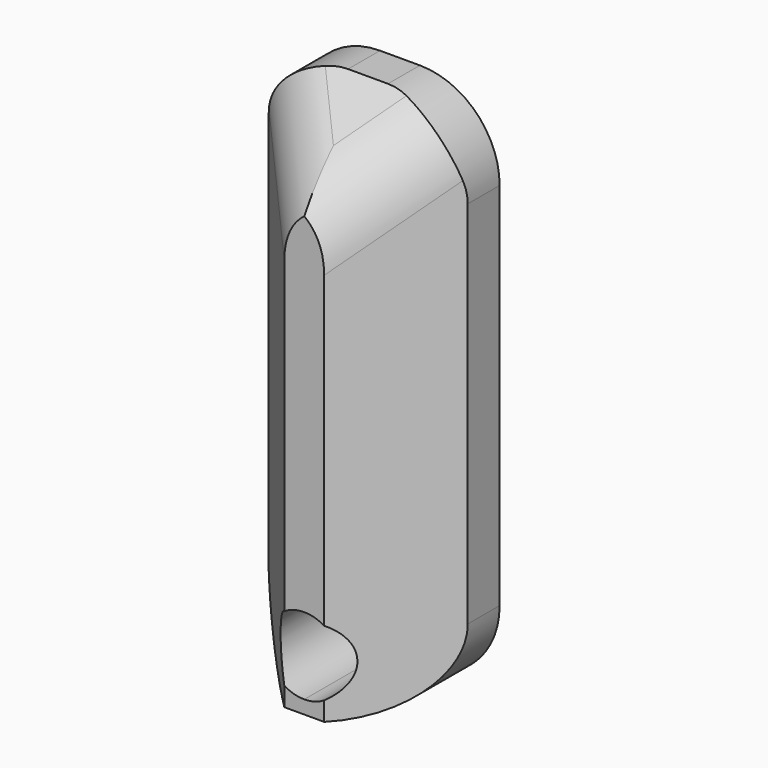
from build123d import *

# Parameters (mm, degrees)
F0_W        = 12.7
F0_H        = 33.7210557661
F1_DEPTH    = 7.62
F3_DEPTH    = 25.4
F4_T1_DEPTH = 59.8493549238
F4_T3_DEPTH = 38.8282991577
F5_T1_DEPTH = 27.94
F5_T3_DEPTH = 23.4635149399
F5_T5_DEPTH = 23.4635149399


# Not quite as in the source:
# - a fillet or chamfer that OpenCascade refuses, or shapes differently, is made with other operations: its cross-section is extruded or revolved along the edge and cut away or added


with BuildPart() as f1:
    # F0 (on Front) → F1 (new body)
    with BuildSketch(Plane.XZ):
        with Locations((-28.5366901662, 2.3533813655)):
            Rectangle(F0_W, F0_H)
    extrude(amount=F1_DEPTH)

    # F2 (on face) → F3 (cut)
    with BuildSketch(Plane.XZ.offset(7.62)):
        with BuildLine():
            ThreePointArc((-28.5366901662, -8.7627890215), (-30.9828768324, -11.2089756876), (-28.5366901662, -13.6551623538))
            Line((-28.5366901662, -13.6551623538), (-28.5366901662, -8.7627890215))
        make_face()
        with BuildLine():
            Line((-28.5366901662, -8.7627890215), (-28.5366901662, -13.6551623538))
            ThreePointArc((-28.5366901662, -13.6551623538), (-26.8069749865, -12.9386908673), (-26.0905035001, -11.2089756876))
            ThreePointArc((-26.0905035001, -11.2089756876), (-26.8069749865, -9.4792605079), (-28.5366901662, -8.7627890215))
        make_face()
    extrude(amount=-F3_DEPTH, mode=Mode.SUBTRACT)

    # F4: chamfer of 5.08 on 3 edges, made by hand

    # F4_s2 → F4_t1 (cut)
    with BuildSketch(Plane.XY.offset(-27.5712960964)):
        Polygon((-22.1866901662, -2.54), (-27.2666901662, -7.62), (-22.1866901662, -7.62), align=None)
        Polygon((-34.8866901662, -2.54), (-29.8066901662, -7.62), (-34.8866901662, -7.62), align=None)
    extrude(amount=F4_T1_DEPTH, mode=Mode.SUBTRACT)

    # F4_s4 → F4_t3 (cut)
    with BuildSketch(Plane.YZ.offset(-47.9508397451)):
        Polygon((-2.54, 19.2139092486), (-7.62, 14.1339092486), (-7.62, 19.2139092486), align=None)
    extrude(amount=F4_T3_DEPTH, mode=Mode.SUBTRACT)

    # F5: fillet of radius 5.08 on 6 edges, made by hand

    # F5_s2 → F5_t1 (cut)
    with BuildSketch(Plane.XZ.offset(-12.7)):
        with BuildLine():
            ThreePointArc((-29.8066901662, 19.2139092486), (-33.3987926146, 17.726011697), (-34.8866901662, 14.1339092486))
            Line((-34.8866901662, 14.1339092486), (-34.8866901662, 19.2139092486))
            Line((-34.8866901662, 19.2139092486), (-29.8066901662, 19.2139092486))
        make_face()
        with BuildLine():
            ThreePointArc((-27.2666901662, 19.2139092486), (-23.6745877178, 17.726011697), (-22.1866901662, 14.1339092486))
            Line((-22.1866901662, 14.1339092486), (-22.1866901662, 19.2139092486))
            Line((-22.1866901662, 19.2139092486), (-27.2666901662, 19.2139092486))
        make_face()
        with BuildLine():
            ThreePointArc((-22.1866901662, -9.4271465175), (-23.6745877178, -13.0192489659), (-27.2666901662, -14.5071465175))
            Line((-27.2666901662, -14.5071465175), (-22.1866901662, -14.5071465175))
            Line((-22.1866901662, -14.5071465175), (-22.1866901662, -9.4271465175))
        make_face()
        with BuildLine():
            ThreePointArc((-34.8866901662, -9.4271465175), (-33.3987926146, -13.0192489659), (-29.8066901662, -14.5071465175))
            Line((-29.8066901662, -14.5071465175), (-34.8866901662, -14.5071465175))
            Line((-34.8866901662, -14.5071465175), (-34.8866901662, -9.4271465175))
        make_face()
    extrude(amount=F5_T1_DEPTH, mode=Mode.SUBTRACT)

    # F5_s4 → F5_t3 (cut)
    with BuildSketch(Plane(origin=(-11.1509269725, -11.1509269725, -11.1509269725), x_dir=(-0.7071067812, 0.7071067812, 0), z_dir=(0.5773502692, 0.5773502692, 0.5773502692))):
        with BuildLine():
            ThreePointArc((16.4323078444, 27.2491898807), (14.5728987932, 25.3897808294), (13.8923078444, 22.8497808294))
            Line((13.8923078444, 22.8497808294), (13.8923078444, 25.7827201969))
            Line((13.8923078444, 25.7827201969), (16.4323078444, 27.2491898807))
        make_face()
    extrude(amount=F5_T3_DEPTH, mode=Mode.SUBTRACT)

    # F5_s6 → F5_t5 (cut)
    with BuildSketch(Plane(origin=(-7.8735331383, 7.8735331383, 7.8735331383), x_dir=(-0.7071067812, -0.7071067812, 0), z_dir=(-0.5773502692, 0.5773502692, 0.5773502692))):
        with BuildLine():
            ThreePointArc((23.9246664139, 3.949079929), (25.7840754651, 2.0896708777), (26.4646664139, -0.4503291223))
            Line((26.4646664139, -0.4503291223), (26.4646664139, 2.4826102452))
            Line((26.4646664139, 2.4826102452), (23.9246664139, 3.949079929))
        make_face()
    extrude(amount=F5_T5_DEPTH, mode=Mode.SUBTRACT)


solid = f1.part
